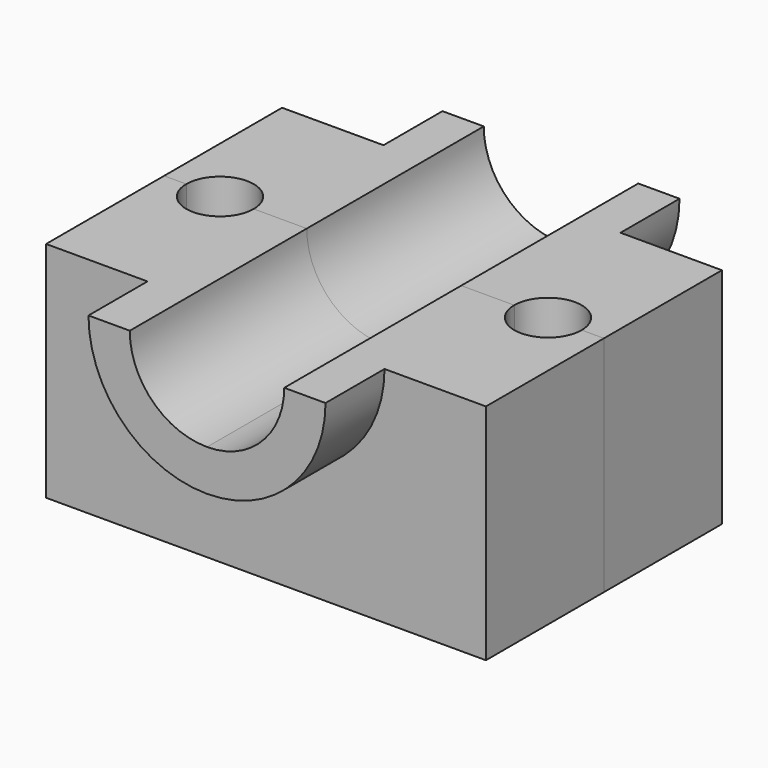
from build123d import *
from build123d import SkipClean  # not in build123d's __all__

# Parameters (mm, degrees)
F1_DEPTH = 25.4
F2_DEPTH = 12.7
F4_DEPTH = 254


with BuildPart() as f1:
    # F0 (on Front) → F1 (new body)
    with BuildSketch(Plane.XZ):
        with BuildLine():
            Line((-37.8727540374, 38.4819693863), (-37.8727540374, 0))
            Line((-37.8727540374, 0), (0, 0))
            Line((0, 0), (0, 18.0733259767))
            ThreePointArc((0, 18.0733259767), (-14.4310901498, 24.0508792366), (-20.4086434096, 38.4819693863))
            Line((-20.4086434096, 38.4819693863), (-37.8727540374, 38.4819693863))
        make_face()
        with BuildLine():
            Line((-13.3011555299, 38.4819693863), (-20.4086434096, 38.4819693863))
            ThreePointArc((-20.4086434096, 38.4819693863), (-14.4310901498, 24.0508792366), (0, 18.0733259767))
            Line((0, 18.0733259767), (0, 25.1808138564))
            ThreePointArc((0, 25.1808138564), (-9.4053372728, 29.0766321135), (-13.3011555299, 38.4819693863))
        make_face()
    extrude(amount=-F1_DEPTH)

    # F0 (on Front) → F2 (join)
    with BuildSketch(Plane.XZ):
        with BuildLine():
            Line((-13.3011555299, 38.4819693863), (-20.4086434096, 38.4819693863))
            ThreePointArc((-20.4086434096, 38.4819693863), (-14.4310901498, 24.0508792366), (0, 18.0733259767))
            Line((0, 18.0733259767), (0, 25.1808138564))
            ThreePointArc((0, 25.1808138564), (-9.4053372728, 29.0766321135), (-13.3011555299, 38.4819693863))
        make_face()
    extrude(amount=F2_DEPTH)

    # F3 (on face) → F4 (cut)
    with BuildSketch(Plane.XY.offset(38.4819693863)):
        with BuildLine():
            ThreePointArc((-34.0433958918, 25.4), (-28.239807114, 19.5964112222), (-22.4362183362, 25.4))
            Line((-22.4362183362, 25.4), (-34.0433958918, 25.4))
        make_face()
    extrude(amount=-F4_DEPTH, mode=Mode.SUBTRACT)

    # F5: F1 across face


with BuildPart() as f1_1:
    add(f1.part, clean=False)
    add(f1.part.mirror(Plane(origin=(0, 10.3439929045, 13.7080154385), x_dir=(0, 1, 0), z_dir=(1, 0, 0))), clean=False)

    # F6: F1 across face


with BuildPart() as f1_2:
    add(f1_1.part, clean=False)
    with SkipClean():  # cleaning this boolean's faces spoils the solid; the shape is the same uncleaned
        add(f1_1.part.mirror(Plane(origin=(0, 25.4, 16.6331926938), x_dir=(-1, 0, 0), z_dir=(0, 1, 0))), clean=False)


solid = f1_2.part
